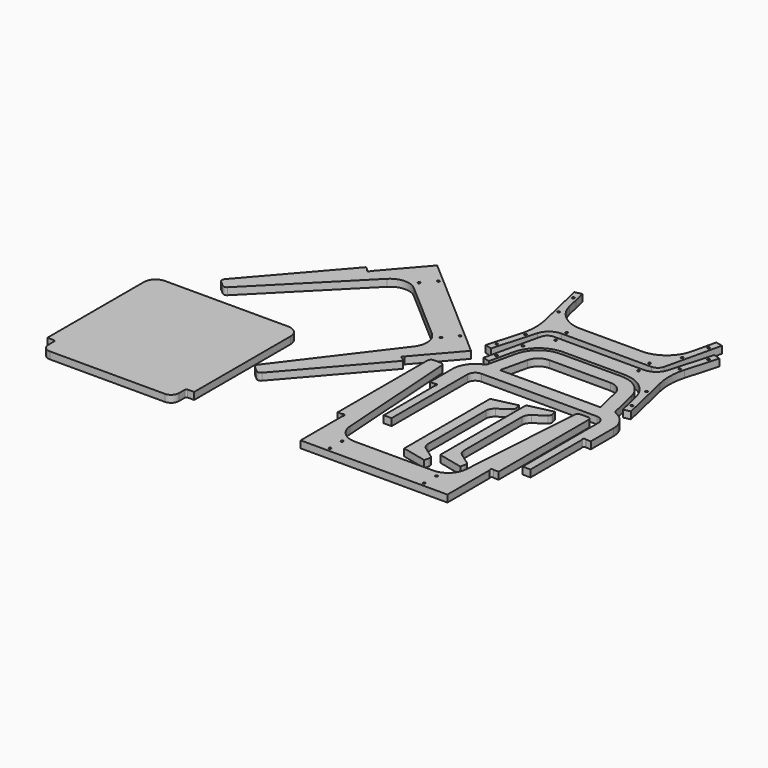
from build123d import *

# Parameters (mm, degrees)
F1_DEPTH = 18
F0_R     = 2.999994


# Not quite as in the source:
# - ends of sketch curves that miss each other by under 0.0002 mm in the source are joined


with BuildPart() as f1:
    # F0 (on Top) → F1 (new body)
    with BuildSketch(Plane.XY):
        with BuildLine():
            Line((-208.1210976, -409.1903424), (-208.1210976, -390.3810582))
            ThreePointArc((-208.1210976, -390.3810582), (-206.9495270679, -387.5526367321), (-204.1211056, -386.3810662))
            Line((-204.1211056, -386.3810662), (-187.6211386, -386.3810662))
            Line((-187.6211386, -386.3810662), (-187.6211386, -79.1910024))
            ThreePointArc((-187.6211386, -79.1910024), (-196.4079175908, -57.9778413908), (-217.6210786, -49.1910624))
            Line((-217.6210786, -49.1910624), (-531.6204506, -49.1910624))
            ThreePointArc((-531.6204506, -49.1910624), (-552.8336116092, -57.9778413908), (-561.6203906, -79.1910024))
            Line((-561.6203906, -79.1910024), (-561.6203906, -386.3810662))
            Line((-561.6203906, -386.3810662), (-545.1204236, -386.3810662))
            ThreePointArc((-545.1204236, -386.3810662), (-542.2920021321, -387.5526367321), (-541.1204316, -390.3810582))
            Line((-541.1204316, -390.3810582), (-541.1204316, -409.1903424))
            ThreePointArc((-541.1204316, -409.1903424), (-535.2625789395, -423.3324497395), (-521.1204716, -429.1903024))
            Line((-521.1204716, -429.1903024), (-228.1210576, -429.1903024))
            ThreePointArc((-228.1210576, -429.1903024), (-213.9789502605, -423.3324497395), (-208.1210976, -409.1903424))
        make_face()
    extrude(amount=F1_DEPTH)


with BuildPart() as f1b:
    # F0 (on Top) → F1, piece 2 (new body)
    with BuildSketch(Plane.XY):
        with BuildLine():
            ThreePointArc((-146.9632314481, -238.4146868251), (-140.4299299166, -240.5974563393), (-134.2667369749, -237.5211656481))
            Line((-134.2667369749, -237.5211656481), (53.2651208, -21.5952578))
            Line((53.2651208, -21.5952578), (43.9460132, -13.501624))
            ThreePointArc((43.9460132, -13.501624), (39.67506775, -9.7922968261), (43.384392922, -5.5213633233))
            Line((43.384392922, -5.5213633233), (131.7403766, 96.2125076))
            Line((131.7403766, 96.2125076), (-150.6302296, 341.4516412))
            Line((-150.6302296, 341.4516412), (-238.9862124, 239.7177578))
            ThreePointArc((-238.9862124, 239.7177578), (-242.6955395739, 235.44683775), (-246.966471298, 239.1561376471))
            Line((-246.966471298, 239.1561376471), (-256.2855682, 247.2497976))
            Line((-256.2855682, 247.2497976), (-443.8174004, 31.3238896))
            ThreePointArc((-443.8174004, 31.3238896), (-446.0001678083, 24.7905858797), (-442.9238519945, 18.6273968789))
            Line((-442.9238519945, 18.6273968789), (-429.6507282, 7.099681))
            ThreePointArc((-429.6507282, 7.099681), (-423.4167045948, 4.9008534233), (-417.3620819773, 7.5540623716))
            Line((-417.3620819773, 7.5540623716), (-192.404746, 234.1626))
            ThreePointArc((-192.404746, 234.1626), (-159.8677433039, 248.4206529084), (-126.366633516, 236.6043944854))
            Line((-126.366633516, 236.6043944854), (-50.9192276, 171.0782456))
            Line((-50.9192276, 171.0782456), (24.5281958, 105.552113))
            ThreePointArc((24.5281958, 105.552113), (40.920134599, 74.0361917378), (31.3597349024, 39.8229283266))
            Line((31.3597349024, 39.8229283266), (-161.5076526, -214.6557556))
            ThreePointArc((-161.5076526, -214.6557556), (-163.2866832453, -221.0223080186), (-160.2364078481, -226.8869222251))
            Line((-160.2364078481, -226.8869222251), (-146.9632314481, -238.4146868251))
        make_face()
        with Locations((-131.9786794, 260.749923)):
            Circle(F0_R, mode=Mode.SUBTRACT)
        with Locations((-106.487468, 290.1007406)):
            Circle(F0_R, mode=Mode.SUBTRACT)
        with Locations((49.2217202, 103.3771872)):
            Circle(F0_R, mode=Mode.SUBTRACT)
        with Locations((74.712957, 132.7280302)):
            Circle(F0_R, mode=Mode.SUBTRACT)
    extrude(amount=F1_DEPTH)


with BuildPart() as f1c:
    # F0 (on Top) → F1, piece 3 (new body)
    with BuildSketch(Plane.XY):
        with BuildLine():
            Line((225.8750626, 266.5747018), (455.3444284, 266.5747018))
            ThreePointArc((455.3444284, 266.5747018), (467.794691029, 270.9225258285), (474.8317877297, 282.075636755))
            Line((474.8317877297, 282.075636755), (507.8610874, 425.1411614))
            Line((507.8610874, 425.1411614), (490.3224382, 429.190277))
            Line((490.3224382, 429.190277), (483.3257675427, 398.8843459837))
            Line((483.3257675427, 398.8843459837), (476.3290956, 368.5784094))
            ThreePointArc((476.3290956, 368.5784094), (448.1807150848, 323.9659333206), (398.3796452, 306.5746218))
            Line((398.3796452, 306.5746218), (320.6399226, 306.5746218))
            Line((320.6399226, 306.5746218), (242.9002, 306.5746218))
            ThreePointArc((242.9002, 306.5746218), (193.0991301152, 323.9659333206), (164.9507515464, 368.5784098494))
            Line((164.9507515464, 368.5784098494), (158.3244350573, 397.2801327837))
            Line((158.3244350573, 397.2801327837), (151.6981218, 425.9818506))
            Line((151.6981218, 425.9818506), (134.1594726, 421.9327858))
            Line((134.1594726, 421.9327858), (164.413946, 290.8863372))
            ThreePointArc((164.413946, 290.8863372), (168.2070122741, 253.2172092865), (162.4476759118, 215.7982237164))
            Line((162.4476759118, 215.7982237164), (138.9987568, 134.0221094))
            Line((138.9987568, 134.0221094), (156.30144, 129.060702))
            Line((156.30144, 129.060702), (187.4246696, 237.6002614))
            ThreePointArc((187.4246696, 237.6002614), (201.8025124395, 258.5201402857), (225.8750626, 266.5747018))
        make_face()
        with Locations((153.2950706, 151.2277646)):
            Circle(F0_R, mode=Mode.SUBTRACT)
        with Locations((172.6073002, 218.5774902)):
            Circle(F0_R, mode=Mode.SUBTRACT)
        with Locations((231.6549596, 276.0746828)):
            Circle(F0_R, mode=Mode.SUBTRACT)
        with Locations((163.2598208, 335.8939688)):
            Circle(F0_R, mode=Mode.SUBTRACT)
        with Locations((148.1233004, 401.4574902)):
            Circle(F0_R, mode=Mode.SUBTRACT)
        with Locations((442.8359952, 276.0746828)):
            Circle(F0_R, mode=Mode.SUBTRACT)
        with Locations((478.0200498, 335.8939688)):
            Circle(F0_R, mode=Mode.SUBTRACT)
        with Locations((493.1565448, 401.4574902)):
            Circle(F0_R, mode=Mode.SUBTRACT)
    extrude(amount=F1_DEPTH)


with BuildPart() as f1d:
    # F0 (on Top) → F1, piece 4 (new body)
    with BuildSketch(Plane.XY):
        with BuildLine():
            Line((451.522465, 246.5887626), (222.0530992, 246.5887626))
            ThreePointArc((222.0530992, 246.5887626), (209.602836571, 242.2409385715), (202.5657398703, 231.087827645))
            Line((202.5657398703, 231.087827645), (169.5364402, 88.0223284))
            Line((169.5364402, 88.0223284), (187.0750894, 83.9731874))
            Line((187.0750894, 83.9731874), (194.0717600573, 114.2791184163))
            Line((194.0717600573, 114.2791184163), (201.068432, 144.585055))
            ThreePointArc((201.068432, 144.585055), (229.2168125152, 189.1975310794), (279.0178824, 206.5888426))
            Line((279.0178824, 206.5888426), (356.757605, 206.5888426))
            Line((356.757605, 206.5888426), (434.4973276, 206.5888426))
            ThreePointArc((434.4973276, 206.5888426), (484.2983974848, 189.1975310794), (512.4467760536, 144.5850545506))
            Line((512.4467760536, 144.5850545506), (519.0730925427, 115.8833316163))
            Line((519.0730925427, 115.8833316163), (525.6994058, 87.1816138))
            Line((525.6994058, 87.1816138), (543.238055, 91.2306786))
            Line((543.238055, 91.2306786), (512.9835816, 222.2771272))
            ThreePointArc((512.9835816, 222.2771272), (509.1905146824, 259.9462559394), (514.9498449582, 297.3652426134))
            Line((514.9498449582, 297.3652426134), (538.3987708, 379.141355))
            Line((538.3987708, 379.141355), (521.0960876, 384.1027878))
            Line((521.0960876, 384.1027878), (489.972858, 275.5632284))
            ThreePointArc((489.972858, 275.5632284), (475.5950249102, 254.6433314613), (451.522465, 246.5887626))
        make_face()
        with Locations((184.2409828, 111.7059742)):
            Circle(F0_R, mode=Mode.SUBTRACT)
        with Locations((199.3774778, 177.269521)):
            Circle(F0_R, mode=Mode.SUBTRACT)
        with Locations((529.2742272, 111.7059742)):
            Circle(F0_R, mode=Mode.SUBTRACT)
        with Locations((514.1377068, 177.269521)):
            Circle(F0_R, mode=Mode.SUBTRACT)
        with Locations((234.5615324, 237.0887816)):
            Circle(F0_R, mode=Mode.SUBTRACT)
        with Locations((445.742568, 237.0887816)):
            Circle(F0_R, mode=Mode.SUBTRACT)
        with Locations((504.7902274, 294.5859996)):
            Circle(F0_R, mode=Mode.SUBTRACT)
        with Locations((524.102457, 361.9356998)):
            Circle(F0_R, mode=Mode.SUBTRACT)
    extrude(amount=F1_DEPTH)


with BuildPart() as f1e:
    # F0 (on Top) → F1, piece 5 (new body)
    with BuildSketch(Plane.XY):
        with BuildLine():
            Line((210.2124574, 142.4720798), (203.2162005008, 112.1679696702))
            Line((203.2162005008, 112.1679696702), (194.523487, 74.5157006))
            ThreePointArc((194.523487, 74.5157006), (191.8167074181, 69.0855468667), (186.9403246174, 65.4752638717))
            ThreePointArc((186.9403246174, 65.4752638717), (161.2502759573, 44.097856598), (151.6211852, 12.0939052))
            Line((151.6211852, 12.0939052), (151.6211852, -59.612911))
            Line((151.6211852, -59.612911), (163.9643152, -59.612911))
            ThreePointArc((163.9643152, -59.612911), (169.6211600179, -59.6129382821), (169.6211536679, -65.2697748679))
            Line((169.6211536679, -65.2697748679), (169.6211492, -229.1815076))
            Line((169.6211492, -229.1815076), (189.6211092, -229.1815076))
            Line((189.6211092, -229.1815076), (189.6211092, 12.0939052))
            ThreePointArc((189.6211092, 12.0939052), (195.4789618605, 26.2360125395), (209.6210692, 32.0938652))
            Line((209.6210692, 32.0938652), (503.6204812, 32.0938652))
            ThreePointArc((503.6204812, 32.0938652), (517.7625885395, 26.2360125395), (523.6204412, 12.0939052))
            Line((523.6204412, 12.0939052), (523.6204412, -229.1815076))
            Line((523.6204412, -229.1815076), (543.6204012, -229.1815076))
            Line((543.6204012, -229.1815076), (543.6204012, -65.2697704))
            ThreePointArc((543.6204012, -65.2697704), (543.6203967321, -59.6129319321), (549.2772396679, -59.6129319321))
            Line((549.2772396679, -59.6129319321), (561.6203652, -59.612911))
            Line((561.6203652, -59.612911), (561.6203652, 12.0939052))
            ThreePointArc((561.6203652, 12.0939052), (551.9912744427, 44.097856598), (526.301228869, 65.4752711359))
            ThreePointArc((526.301228869, 65.4752711359), (521.4248590341, 69.0855580108), (518.7180781382, 74.5157040026))
            Line((518.7180781382, 74.5157040026), (503.029093, 142.4720798))
            ThreePointArc((503.029093, 142.4720798), (478.2321270638, 181.7728790581), (434.3604978, 197.0935352))
            Line((434.3604978, 197.0935352), (356.757605, 197.0935352))
            Line((356.757605, 197.0935352), (278.8810526, 197.0935352))
            ThreePointArc((278.8810526, 197.0935352), (235.0094233362, 181.7728790581), (210.2124574, 142.4720798))
        make_face()
        with BuildLine():
            ThreePointArc((434.3604978, 162.0936052), (456.4441656009, 154.3816425892), (468.9262136401, 134.5987907322))
            Line((468.9262136401, 134.5987907322), (484.510969, 67.0937952))
            Line((484.510969, 67.0937952), (228.7305814, 67.0937952))
            Line((228.7305814, 67.0937952), (244.315361, 134.598791))
            ThreePointArc((244.315361, 134.598791), (256.7973870349, 154.3816443677), (278.8810526, 162.0936052))
            Line((278.8810526, 162.0936052), (434.3604978, 162.0936052))
        make_face(mode=Mode.SUBTRACT)
    extrude(amount=F1_DEPTH)


with BuildPart() as f1f:
    # F0 (on Top) → F1, piece 6 (new body)
    with BuildSketch(Plane.XY):
        with BuildLine():
            Line((500.0409862, -276.498431), (500.0409862, 9.4948756))
            ThreePointArc((500.0409862, 9.4948756), (497.4049525028, 15.8588239028), (491.0410042, 18.4948576))
            Line((491.0410042, 18.4948576), (473.460699, 18.4948576))
            ThreePointArc((473.460699, 18.4948576), (467.3121785267, 16.067194216), (464.4806731361, 10.0938843512))
            Line((464.4806731361, 10.0938843512), (443.2291618, -308.5055552))
            ThreePointArc((443.2291618, -308.5055552), (428.0129103297, -340.6056254582), (394.9712954, -353.651693))
            Line((394.9712954, -353.651693), (295.0413962, -353.651693))
            Line((295.0413962, -353.651693), (195.1114716, -353.6517184))
            ThreePointArc((195.1114716, -353.6517184), (162.0698572875, -340.6056260357), (146.8536291716, -308.5055552953))
            Line((146.8536291716, -308.5055552953), (125.6020856, 10.0938838))
            ThreePointArc((125.6020856, 10.0938838), (122.7705884733, 16.067194216), (116.622068, 18.4948576))
            Line((116.622068, 18.4948576), (99.041839, 18.4948576))
            ThreePointArc((99.041839, 18.4948576), (92.6778906972, 15.8588239028), (90.041857, 9.4948756))
            Line((90.041857, 9.4948756), (90.041857, -276.498431))
            Line((90.041857, -276.498431), (102.384987, -276.498431))
            ThreePointArc((102.384987, -276.498431), (108.0418318179, -276.4984328821), (108.0418127679, -282.1552821678))
            Line((108.0418127679, -282.1552821678), (108.041821, -416.9015792))
            Line((108.041821, -416.9015792), (482.0410222, -416.9015792))
            Line((482.0410222, -416.9015792), (482.0410222, -282.1552904))
            ThreePointArc((482.0410222, -282.1552904), (482.0410113821, -276.4984328821), (487.6978606679, -276.4984265321))
            Line((487.6978606679, -276.4984265321), (500.0409862, -276.498431))
        make_face()
        with Locations((175.0416362, -407.0768084)):
            Circle(F0_R, mode=Mode.SUBTRACT)
        with Locations((175.0416362, -368.2017274)):
            Circle(F0_R, mode=Mode.SUBTRACT)
        with Locations((415.0411562, -407.0768084)):
            Circle(F0_R, mode=Mode.SUBTRACT)
        with Locations((415.0411562, -368.2017274)):
            Circle(F0_R, mode=Mode.SUBTRACT)
    extrude(amount=F1_DEPTH)


with BuildPart() as f1g:
    # F0 (on Top) → F1, piece 7 (new body)
    with BuildSketch(Plane.XY):
        with BuildLine():
            Line((426.447077, -4.285107), (363.9428332, -18.715355))
            Line((363.9428332, -18.715355), (363.9428332, -292.0261114))
            Line((363.9428332, -292.0261114), (426.447077, -306.4563848))
            Line((426.447077, -306.4563848), (429.2000306, -294.5320754))
            ThreePointArc((429.2000306, -294.5320754), (428.8247730466, -289.0692647459), (425.4695209139, -284.7419816178))
            Line((425.4695209139, -284.7419816178), (398.3567852, -265.5584224))
            ThreePointArc((398.3567852, -265.5584224), (391.4357290231, -257.6076055326), (388.9428086, -247.3654438))
            Line((388.9428086, -247.3654438), (388.9428086, -63.3760734))
            ThreePointArc((388.9428086, -63.3760734), (391.4357323943, -53.1339051525), (398.3567946587, -45.1830827683))
            Line((398.3567946587, -45.1830827683), (425.4695072, -25.9994908))
            ThreePointArc((425.4695072, -25.9994908), (428.8247730466, -21.6722270541), (429.2000237777, -16.2094179751))
            Line((429.2000237777, -16.2094179751), (426.447077, -4.285107))
        make_face()
    extrude(amount=F1_DEPTH)


with BuildPart() as f1h:
    # F0 (on Top) → F1, piece 8 (new body)
    with BuildSketch(Plane.XY):
        with BuildLine():
            Line((353.1833424, -27.4380198), (290.6790986, -41.8682932))
            Line((290.6790986, -41.8682932), (290.6790986, -315.1790242))
            Line((290.6790986, -315.1790242), (353.1833424, -329.6092976))
            Line((353.1833424, -329.6092976), (355.936296, -317.6849882))
            ThreePointArc((355.936296, -317.6849882), (355.5610314284, -312.2221845279), (352.2057743377, -307.8949113441))
            Line((352.2057743377, -307.8949113441), (325.093076, -288.7113352))
            ThreePointArc((325.093076, -288.7113352), (318.1719991877, -280.7605275403), (315.679074, -270.5183566))
            Line((315.679074, -270.5183566), (315.679074, -86.5289862))
            ThreePointArc((315.679074, -86.5289862), (318.1719991877, -76.2868152597), (325.0930650088, -68.3359920658))
            Line((325.0930650088, -68.3359920658), (352.2057726, -49.152429))
            ThreePointArc((352.2057726, -49.152429), (355.5610314284, -44.8251582721), (355.936294745, -39.3623548897))
            Line((355.936294745, -39.3623548897), (353.1833424, -27.4380198))
        make_face()
    extrude(amount=F1_DEPTH)


solid = Compound([f1.part, f1b.part, f1c.part, f1d.part, f1e.part, f1f.part, f1g.part, f1h.part])
